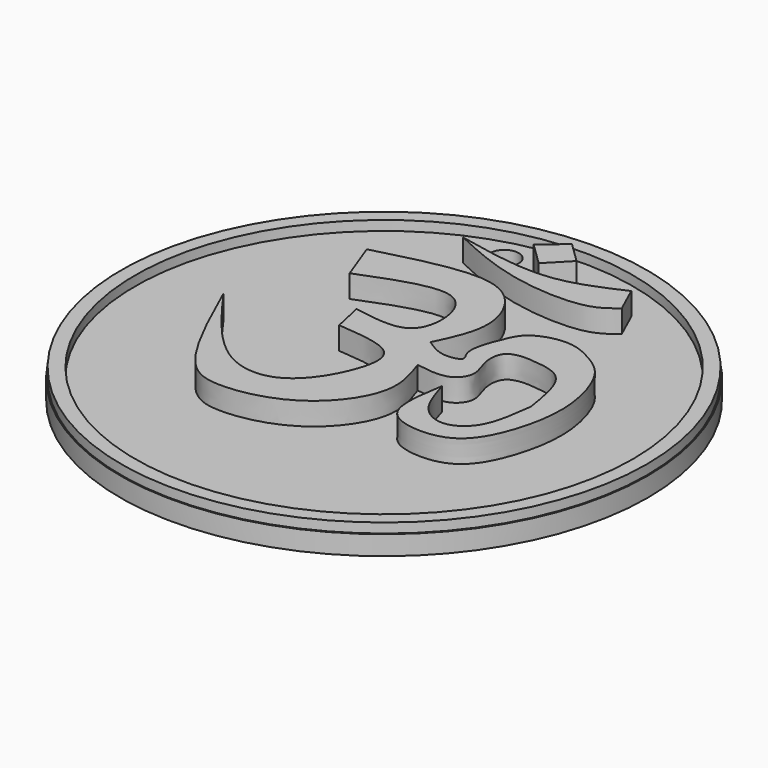
from build123d import *

# Parameters (mm, degrees)
F0_R     = 40.8737100338
F1_DEPTH = 3
F2_R     = 40.6957539797
F2_R_2   = 38.5419315624
F3_DEPTH = 1.5
F5_DEPTH = 3.5
F6_R     = 2.1975710884
F7_DEPTH = 3


with BuildPart() as f1:
    # F0 (on Top) → F1 (new body)
    with BuildSketch(Plane.XY):
        Circle(F0_R)
    extrude(amount=F1_DEPTH)

    # F2 (on face) → F3 (join)
    with BuildSketch(Plane.XY.offset(3)):
        Circle(F2_R)
        Circle(F2_R_2, mode=Mode.SUBTRACT)
    extrude(amount=F3_DEPTH)

    # F4 (on face) → F5 (join)
    with BuildSketch(Plane.XY.offset(3)):
        with BuildLine():
            add(Edge.make_bspline(
                [(-18.5161922127, 19.791925326), (-12.7151925876, 21.3351674452), (-3.2277425118, 23.859117369), (3.4150540296, 20.4339539585), (6.2694455573, 13.0889481493), (3.9197467048, 8.1734523404), (2.6966251899, 5.6147207506)],
                knots=[0, 0, 0, 0, 0.332446594, 0.5437115441, 0.7624818062, 1, 1, 1, 1], degree=3))
            Line((-18.5161922127, 19.791925326), (-16.20740816, 13.5870669037))
            add(Edge.make_bspline(
                [(-16.20740816, 13.5870669037), (-11.0929458702, 15.6161362843), (-2.752055686, 18.9252319275), (0.6709459709, 12.4764702332), (-0.5376493129, 5.2281596847), (-6.4609189943, 6.24601212), (-9.7139514983, 6.8050120026)],
                knots=[0, 0, 0, 0, 0.3275893752, 0.5342471699, 0.7442106849, 1, 1, 1, 1], degree=3))
            Line((-9.7139514983, 6.8050120026), (-8.7038585916, 2.1874438971))
            add(Edge.make_bspline(
                [(-8.7038585916, 2.1874438971), (-5.0516756353, 1.8971066874), (1.4743799313, 1.3783055249), (0.4320748866, -6.0037109711), (-4.6539335606, -14.2800911607), (-14.7593699815, -14.073892468), (-21.0811542832, -5.254384585), (-24.8474739492, 0)],
                knots=[0, 0, 0, 0, 0.1955278639, 0.3493871254, 0.5461884526, 0.7296333955, 1, 1, 1, 1], degree=3))
            add(Edge.make_bspline(
                [(-24.8474739492, 0), (-21.8108523669, -6.8272496265), (-17.0623369266, -17.5033577248), (-10.2515605655, -19.7180403086), (0.7822052269, -17.4220041674), (7.8494428689, -7.7477839242), (6.0306062721, -2.4276731034), (5.2006347105, 0)],
                knots=[0, 0, 0, 0, 0.2707643094, 0.4234075499, 0.6256267457, 0.8291659872, 1, 1, 1, 1], degree=3))
            add(Edge.make_bspline(
                [(5.2006347105, 0), (7.0558782543, -0.288731548), (10.3259106837, -0.7976466868), (12.5781414282, 2.3991075178), (10.8457845725, 5.4428405295), (11.0488135588, 9.7583543287), (16.3784916805, 9.6098216805), (21.4125144717, 8.4677573473), (22.2506321534, 3.0756632517), (22.7286964655, 0)],
                knots=[0, 0, 0, 0, 0.1522720518, 0.2683930901, 0.393191332, 0.517267269, 0.6610905311, 0.8066852357, 1, 1, 1, 1], degree=3))
            add(Edge.make_bspline(
                [(22.7286964655, 0), (22.3751428346, -2.8940459342), (21.760112666, -7.9284322424), (17.1960973157, -10.7354530989), (12.7814342968, -8.5747040819), (11.6223696105, -4.6521009952), (10.9791178256, -2.475154819)],
                knots=[0, 0, 0, 0, 0.2987774731, 0.5197433814, 0.7334696409, 1, 1, 1, 1], degree=3))
            add(Edge.make_bspline(
                [(10.9791178256, -2.475154819), (10.4143752119, -5.868762178), (9.4170665506, -11.8617117622), (15.7194742185, -13.7352738113), (22.208604559, -12.607886853), (25.7160244182, -4.5211657639), (26.6477559678, 3.6676927283), (24.0516080161, 11.6963261383), (20.3404842083, 14.366500869), (15.9475940403, 16.4684038367), (10.5274427232, 14.8383861124), (9.0509264503, 11.7721150129), (7.1117466969, 6.480918156), (9.3180739858, 4.40547596), (5.5607718644, 3.6452011728), (3.704177681, 4.9218811085), (2.6966251899, 5.6147207506)],
                knots=[0, 0, 0, 0, 0.0927466913, 0.1637862563, 0.2408254215, 0.3302072886, 0.4224188469, 0.511065812, 0.5768972077, 0.6451241214, 0.7155702479, 0.7742736226, 0.8469858668, 0.8895704824, 0.9400711601, 1, 1, 1, 1], degree=3))
        make_face()
        with BuildLine():
            add(Edge.make_bspline(
                [(-11.3643482327, 29.4991154224), (-6.404904251, 28.4573434012), (2.8845705426, 26.5060127748), (9.9821642335, 29.7299226682), (13.2905105129, 31.2326587737)],
                knots=[0, 0, 0, 0, 0.5338777586, 1, 1, 1, 1], degree=3))
            add(Edge.make_bspline(
                [(-11.3643482327, 29.4991154224), (-7.7798241077, 27.8488746747), (-0.6953090811, 24.5873105264), (11.6043928769, 23.9693963536), (14.2279842551, 26.1669657789), (15.2166699991, 26.9951075315)],
                knots=[0, 0, 0, 0, 0.3895762705, 0.76996523, 1, 1, 1, 1], degree=3))
            Line((15.2166699991, 26.9951075315), (13.2905105129, 31.2326587737))
        make_face()
        Polygon((0, 36.3618300318), (-3.4969905391, 33.3261489868), (0, 29.9247764051), (3.2172903236, 33.232509843), align=None)
    extrude(amount=F5_DEPTH)

    # F6 (on face) → F7 (cut)
    with BuildSketch(Plane.XY.offset(3)):
        with Locations((-8.2511557266, 33.6113274097)):
            Circle(F6_R)
    extrude(amount=-F7_DEPTH, mode=Mode.SUBTRACT)


solid = f1.part
